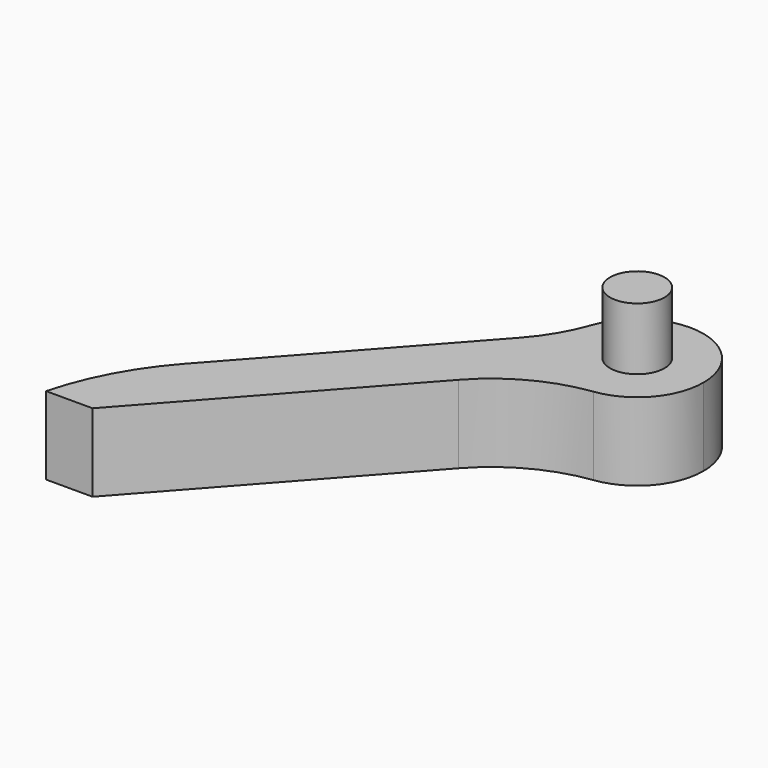
from build123d import *

# Parameters (mm, degrees)
F0_R        = 1.75
F1_DEPTH    = 5
F2_DEPTH    = 9
F3_T1_DEPTH = 31.689764736
F4_R        = 9.8818743841


# Not quite as in the source:
# - a fillet or chamfer that OpenCascade refuses, or shapes differently, is made with other operations: its cross-section is extruded or revolved along the edge and cut away or added


with BuildPart() as f1:
    # F0 (on Top) → F1 (new body)
    with BuildSketch(Plane.XY):
        with BuildLine():
            ThreePointArc((10.3788942671, 7.8619225196), (14.645060229, 7.8336341982), (16.7863510811, 11.523599744))
            ThreePointArc((16.7863510811, 11.523599744), (12.5363510811, 15.773599744), (8.2863510811, 11.523599744))
            ThreePointArc((8.2863510811, 11.523599744), (8.8463855352, 9.4148905962), (10.3788942671, 7.8619225196))
        make_face()
        with Locations((12.5363510811, 11.523599744)):
            Circle(F0_R, mode=Mode.SUBTRACT)
        with BuildLine():
            ThreePointArc((10.3788942671, 7.8619225196), (8.8463855352, 9.4148905962), (8.2863510811, 11.523599744))
            Line((8.2863510811, 11.523599744), (-8.3690416068, -7.120377686))
            Line((-8.3690416068, -7.120377686), (-5.386005218, -9.7852405161))
            Line((-5.386005218, -9.7852405161), (10.3788942671, 7.8619225196))
        make_face()
        Polygon((-5.386005218, -9.7852405161), (-8.3690416068, -7.120377686), (-8.3690416068, -9.7852405161), align=None)
    extrude(amount=F1_DEPTH)

    # F0 (on Top) → F2 (join)
    with BuildSketch(Plane.XY):
        with Locations((12.5363510811, 11.523599744)):
            Circle(F0_R)
    extrude(amount=F2_DEPTH)

    # F3: fillet of radius 16 on 1 edges, made by hand

    # F3_s2 → F3_t1 (cut)
    with BuildSketch(Plane.XY.offset(-13.344882368)):
        with BuildLine():
            ThreePointArc((-4.8128135074, -3.1395507152), (-6.9878475663, -6.2499965822), (-8.3690416068, -9.7852405161))
            Line((-8.3690416068, -9.7852405161), (-8.3690416068, -7.120377686))
            Line((-8.3690416068, -7.120377686), (-4.8128135074, -3.1395507152))
        make_face()
    extrude(amount=F3_T1_DEPTH, mode=Mode.SUBTRACT)

    # F4
    f4_edges = [f1.edges().sort_by_distance(p)[0] for p in [
        (8.286351, 11.5236, 2.5),
        (10.378894, 7.861923, 2.5),
    ]]
    fillet(f4_edges, radius=F4_R)


solid = f1.part
